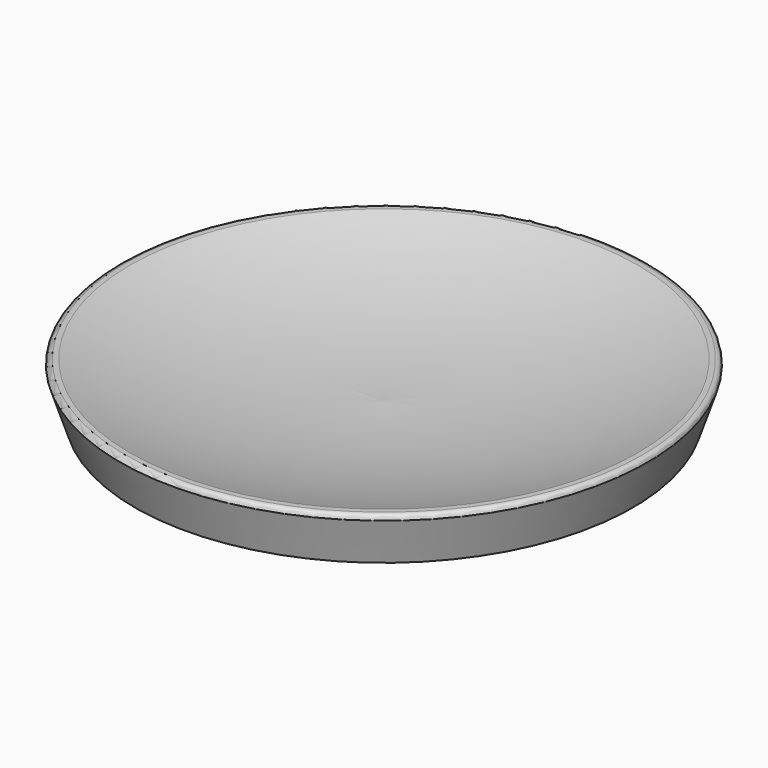
from build123d import *

# Parameters (mm, degrees)
F2_SIZE2 = 9
F2_SIZE  = 3
F3_R     = 0.99999


# Not quite as in the source:
# - a fillet or chamfer is up to 0.001 mm smaller than in the source, because OpenCascade refuses the exact size


with BuildPart() as f1:
    # F0 (on Front) → F1 (revolve)
    with BuildSketch(Plane.XZ):
        with BuildLine():
            Line((-53, 0), (0, 0))
            Line((0, 0), (0, 2.5))
            ThreePointArc((0, 2.5), (-25.8481665636, 3.8824673673), (-51, 10))
            Line((-51, 10), (-53, 10))
            Line((-53, 10), (-53, 0))
        make_face()
    revolve(axis=Axis((0, 0, 5), (0, 0, 1)))

    # F2
    f2_edges = [f1.edges().sort_by_distance(p)[0] for p in [
        (53, 0, 0),
    ]]
    f2_side = f1.faces().sort_by_distance((0, 0, 0))[0]
    chamfer(f2_edges, length=F2_SIZE, length2=F2_SIZE2, reference=f2_side)

    # F3 (radius 1 in the source; OpenCascade refuses exactly that, so slightly less here)
    f3_edges = [f1.edges().sort_by_distance(p)[0] for p in [
        (53, 0, 10),
    ]]
    fillet(f3_edges, radius=F3_R)


solid = f1.part
